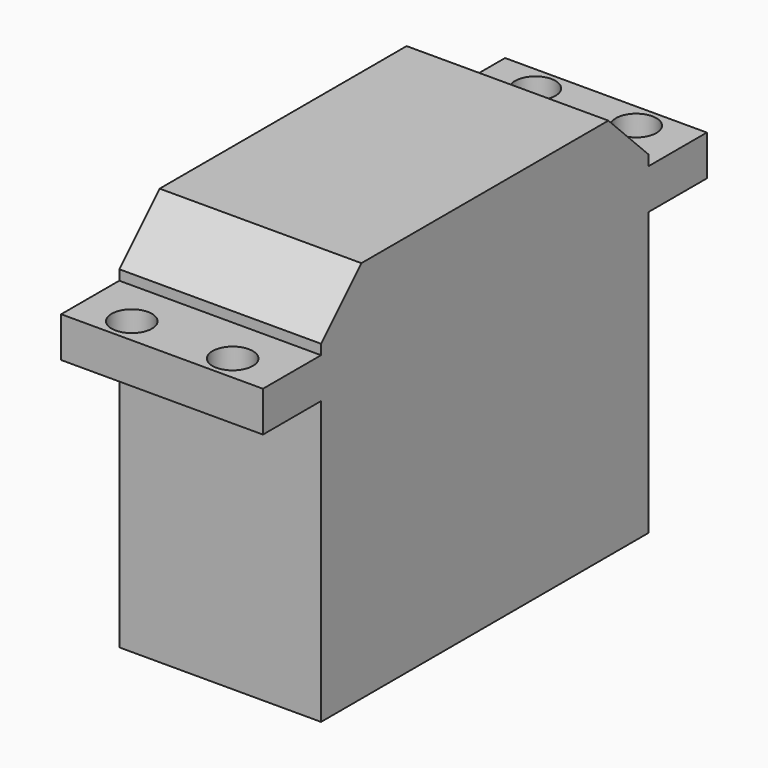
from build123d import *

# Parameters (mm, degrees)
F0_W     = 7.2
F0_H     = 4
F0_W_2   = 40.6
F0_H_2   = 6
F0_H_3   = 28
F1_DEPTH = 10
F3_D     = 4
F4_SIZE  = 5


# Not quite as in the source:
# - the program builds the solid bodies; features that only make, move or delete a surface that nothing else refers to are left out


with BuildPart() as f1:
    # F0 (on Right) → F1 (new body, symmetric)
    with BuildSketch(Plane.YZ):
        with Locations((23.9, 9.8437508568)):
            Rectangle(F0_W, F0_H)
        with Locations((0, 14.8437508568)):
            Rectangle(F0_W_2, F0_H_2)
        with Locations((0, -6.1562491432)):
            Rectangle(F0_W_2, F0_H_3)
        with Locations((-23.9, 9.8437508568)):
            Rectangle(F0_W, F0_H)
        with Locations((0, 9.8437508568)):
            Rectangle(F0_W_2, F0_H)
    extrude(amount=F1_DEPTH, both=True)

    # F3 (through all)
    with Locations(Plane(origin=(0, 0, 0), x_dir=(1, 0, 0), z_dir=(0, 0, -1))):
        with Locations((-5, -25), (5, -25), (5, 25), (-5, 25)):
            Hole(F3_D / 2)

    # F4
    f4_edges = [f1.edges().sort_by_distance(p)[0] for p in [
        (0, -20.3, 17.843751),
        (0, 20.3, 17.843751),
    ]]
    chamfer(f4_edges, length=F4_SIZE)


solid = f1.part
